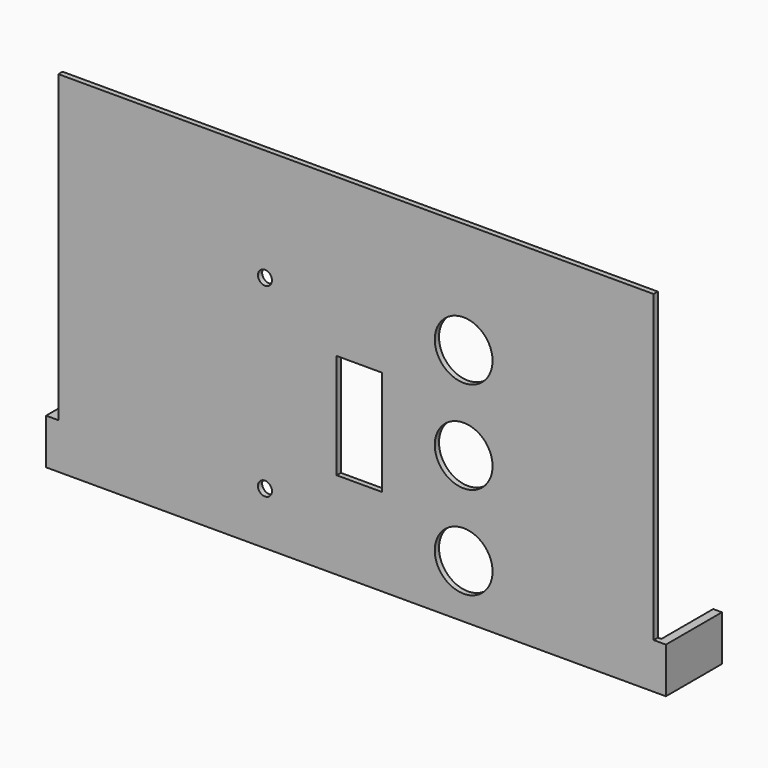
from build123d import *

# Parameters (mm, degrees)
F0_W     = 170
F0_H     = 100
F1_DEPTH = 1.5
F2_R     = 8.25
F2_W     = 13
F2_H     = 30
F2_R_2   = 2
F3_DEPTH = 25
F4_W     = 20
F4_H     = 13
F5_DEPTH = 3.5
F6_W     = 18.5
F6_H     = 13
F7_DEPTH = 1


# Not quite as in the source:
# - a pattern or mirror of a feature is missing from the dataset's text; its kind, count and spacing are read off the source's solid


with BuildPart() as f1:
    # F0 (on Front) → F1 (new body)
    with BuildSketch(Plane.XZ):
        Rectangle(F0_W, F0_H)
    extrude(amount=F1_DEPTH)

    # F2 (on face) → F3 (cut)
    with BuildSketch(Plane.XZ.offset(1.5)):
        with Locations((30.75, -34.75)):
            Circle(F2_R)
        with Locations((30.75, -8.25)):
            Circle(F2_R)
        with Locations((30.75, 18.25)):
            Circle(F2_R)
        with Locations((1, -10)):
            Rectangle(F2_W, F2_H)
        with Locations((-26, -35)):
            Circle(F2_R_2)
        with Locations((-26, 18)):
            Circle(F2_R_2)
    extrude(amount=-F3_DEPTH, mode=Mode.SUBTRACT)

    # F4 (on face) → F5 (join)
    with BuildSketch(Plane.YZ.offset(85)):
        with Locations((8.5, -43.5)):
            Rectangle(F4_W, F4_H)
    f5 = extrude(amount=F5_DEPTH)

    # F5_copies: F5 across plane
    add(f5.mirror(Plane(origin=(0, 0, 0), x_dir=(0, 0, -1), z_dir=(-1, 0, 0))))

    # F6 (on face) → F7 (cut)
    with BuildSketch(Plane(origin=(85, 0, 0), x_dir=(0, -1, 0), z_dir=(-1, 0, 0))):
        with Locations((-9.25, -43.5)):
            Rectangle(F6_W, F6_H)
    f7 = extrude(amount=-F7_DEPTH, mode=Mode.SUBTRACT)

    # F7_copies: F7 across plane
    add(f7.mirror(Plane(origin=(0, 0, 0), x_dir=(0, 0, -1), z_dir=(-1, 0, 0))), mode=Mode.SUBTRACT)


solid = f1.part
